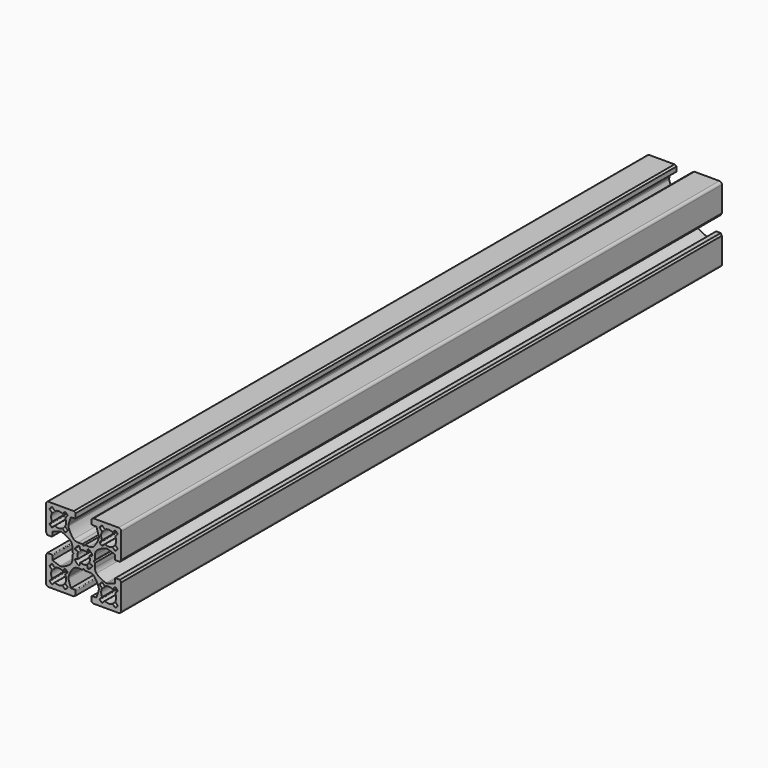
from build123d import *

# Parameters (mm, degrees)
F1_DEPTH = 300


# Not quite as in the source:
# - ends of sketch curves that miss each other by under 0.0002 mm in the source are joined


with BuildPart() as f1:
    # F0 (on Front) → F1 (new body)
    with BuildSketch(Plane.XZ):
        with BuildLine():
            Line((-10.317882, -28.053804), (-8.817882, -28.053804))
            Line((-8.817882, -28.053804), (-8.317882, -27.553804))
            Line((-8.317882, -27.553804), (-8.317882, -25.835963))
            ThreePointArc((-8.317882, -25.835963), (-8.1666472628, -24.8954650055), (-7.7281910149, -24.049790989))
            ThreePointArc((-7.7281910149, -24.049790989), (-5.9278016138, -22.7791417483), (-3.8900220756, -21.9404487353))
            ThreePointArc((-3.8900220756, -21.9404487353), (-3.6281322729, -21.9188378518), (-3.3696549943, -21.9661959825))
            Line((-3.3696549943, -21.9661959825), (-0.317882, -22.953804))
            Line((-0.317882, -22.953804), (-0.317882, -24.603804))
            ThreePointArc((-0.317882, -24.603804), (-0.2300140344, -24.8159360344), (-0.017882, -24.903804))
            Line((-0.017882, -24.903804), (1.682118, -24.903804))
            Line((1.682118, -24.903804), (2.182118, -24.103804))
            Line((2.182118, -24.103804), (2.182118, -14.053804))
            ThreePointArc((2.182118, -14.053804), (1.8892247812, -13.3466972188), (1.182118, -13.053804))
            Line((1.182118, -13.053804), (-8.867882, -13.053804))
            Line((-8.867882, -13.053804), (-9.667882, -13.553804))
            Line((-9.667882, -13.553804), (-9.667882, -15.253804))
            ThreePointArc((-9.667882, -15.253804), (-9.5800140344, -15.4659360344), (-9.367882, -15.553804))
            Line((-9.367882, -15.553804), (-7.717882, -15.553804))
            Line((-7.717882, -15.553804), (-6.730274, -18.605577))
            ThreePointArc((-6.730274, -18.605577), (-6.6829159047, -18.8640542036), (-6.7045263914, -19.1259439149))
            ThreePointArc((-6.7045263914, -19.1259439149), (-7.5432189083, -21.1637239049), (-8.8138685119, -22.9641134339))
            ThreePointArc((-8.8138685119, -22.9641134339), (-9.6595430055, -23.4025692628), (-10.600041, -23.553804))
            Line((-10.600041, -23.553804), (-12.317882, -23.553804))
            Line((-12.317882, -23.553804), (-12.817882, -24.053804))
            Line((-12.817882, -24.053804), (-12.817882, -25.553804))
            ThreePointArc((-12.817882, -25.553804), (-12.2892723342, -25.6103286428), (-11.7845662465, -25.777346543))
            ThreePointArc((-11.7845662465, -25.777346543), (-11.521192295, -25.7698304515), (-11.3653270693, -25.5573959875))
            Line((-11.3653270693, -25.5573959875), (-11.231756, -24.816462))
            ThreePointArc((-11.231756, -24.816462), (-11.061392872, -24.5969122529), (-10.7838767336, -24.6114195492))
            ThreePointArc((-10.7838767336, -24.6114195492), (-9.990624391, -25.2265473595), (-9.3754974572, -26.0198002702))
            ThreePointArc((-9.3754974572, -26.0198002702), (-9.3609903588, -26.2973161033), (-9.5805400125, -26.4676789307))
            Line((-9.5805400125, -26.4676789307), (-10.321473, -26.601249))
            ThreePointArc((-10.321473, -26.601249), (-10.5339073555, -26.757114112), (-10.5414238716, -27.0204879417))
            ThreePointArc((-10.5414238716, -27.0204879417), (-10.3744066428, -27.5251943342), (-10.317882, -28.053804))
        make_face()
        with BuildLine():
            ThreePointArc((-5.5627339656, -19.7356560344), (-5.4787894201, -19.5718836819), (-5.5062620121, -19.389913006))
            ThreePointArc((-5.5062620121, -19.389913006), (-5.820221, -18.053804), (-5.5062614757, -16.7176952608))
            ThreePointArc((-5.5062614757, -16.7176952608), (-5.4787894201, -16.5357243181), (-5.5627339656, -16.3719519656))
            Line((-5.5627339656, -16.3719519656), (-6.303305, -15.631381))
            ThreePointArc((-6.303305, -15.631381), (-6.3907399595, -15.4353436467), (-6.3248118511, -15.2310671199))
            ThreePointArc((-6.3248118511, -15.2310671199), (-6.0022020125, -14.8718239818), (-5.6429589383, -14.5492140766))
            ThreePointArc((-5.6429589383, -14.5492140766), (-5.4386817022, -14.4832850218), (-5.2426439656, -14.5707209656))
            Line((-5.2426439656, -14.5707209656), (-4.502074, -15.311292))
            ThreePointArc((-4.502074, -15.311292), (-4.3383016819, -15.3952365799), (-4.156331006, -15.3677639879))
            ThreePointArc((-4.156331006, -15.3677639879), (-2.8202214477, -15.053804), (-1.484111862, -15.3677637227))
            ThreePointArc((-1.484111862, -15.3677637227), (-1.3021413181, -15.3952365799), (-1.1383689656, -15.3112920344))
            Line((-1.1383689656, -15.3112920344), (-0.397799, -14.570721))
            ThreePointArc((-0.397799, -14.570721), (-0.2017612978, -14.4832850218), (0.0025159751, -14.5492140309))
            ThreePointArc((0.0025159751, -14.5492140309), (0.3617595153, -14.8718234847), (0.684369412, -15.2310666682))
            ThreePointArc((0.684369412, -15.2310666682), (0.7502979573, -15.4353436866), (0.6628620344, -15.6313810344))
            Line((0.6628620344, -15.6313810344), (-0.077709, -16.371952))
            ThreePointArc((-0.077709, -16.371952), (-0.1616535799, -16.5357243181), (-0.1341809879, -16.717694994))
            ThreePointArc((-0.1341809879, -16.717694994), (0.179779, -18.053804), (-0.1341807227, -19.389913138))
            ThreePointArc((-0.1341807227, -19.389913138), (-0.1616535799, -19.5718836819), (-0.0777090344, -19.7356560344))
            Line((-0.0777090344, -19.7356560344), (0.662862, -20.476227))
            ThreePointArc((0.662862, -20.476227), (0.7502979573, -20.6722643134), (0.6843694576, -20.8765413686))
            ThreePointArc((0.6843694576, -20.8765413686), (0.3617595153, -21.2357845153), (0.0025163318, -21.558394412))
            ThreePointArc((0.0025163318, -21.558394412), (-0.2017612978, -21.6243229782), (-0.3977990344, -21.5368870344))
            Line((-0.3977990344, -21.5368870344), (-1.138369, -20.796316))
            ThreePointArc((-1.138369, -20.796316), (-1.3021413181, -20.7123714201), (-1.484111994, -20.7398440121))
            ThreePointArc((-1.484111994, -20.7398440121), (-2.8202214477, -21.053804), (-4.1563309396, -20.7398438786))
            ThreePointArc((-4.1563309396, -20.7398438786), (-4.3383016819, -20.7123714201), (-4.5020740344, -20.7963159656))
            Line((-4.5020740344, -20.7963159656), (-5.242644, -21.536887))
            ThreePointArc((-5.242644, -21.536887), (-5.4386817022, -21.6243229782), (-5.6429589751, -21.5583939691))
            ThreePointArc((-5.6429589751, -21.5583939691), (-6.0022020125, -21.2357840182), (-6.3248118054, -20.8765408433))
            ThreePointArc((-6.3248118054, -20.8765408433), (-6.3907399595, -20.6722643533), (-6.3033045344, -20.4762274656))
            Line((-6.3033045344, -20.4762274656), (-5.5627339656, -19.7356560344))
        make_face(mode=Mode.SUBTRACT)
        with BuildLine():
            Line((-16.817882, -28.053804), (-15.317882, -28.053804))
            ThreePointArc((-15.317882, -28.053804), (-15.2613573135, -27.5251941322), (-15.0943392862, -27.0204878701))
            ThreePointArc((-15.0943392862, -27.0204878701), (-15.1018556445, -26.757114112), (-15.3142900125, -26.6012490693))
            Line((-15.3142900125, -26.6012490693), (-16.055223, -26.467679))
            ThreePointArc((-16.055223, -26.467679), (-16.2747726412, -26.2973161033), (-16.2602657097, -26.0198001716))
            ThreePointArc((-16.2602657097, -26.0198001716), (-15.6451391247, -25.2265468753), (-14.8518861678, -24.611419716))
            ThreePointArc((-14.8518861678, -24.611419716), (-14.574370128, -24.5969122529), (-14.4040070693, -24.8164620125))
            Line((-14.4040070693, -24.8164620125), (-14.270436, -25.557396))
            ThreePointArc((-14.270436, -25.557396), (-14.114570705, -25.7698304515), (-13.8511966819, -25.7773467007))
            ThreePointArc((-13.8511966819, -25.7773467007), (-13.3464912208, -25.6103285465), (-12.817882, -25.553804))
            Line((-12.817882, -25.553804), (-12.817882, -24.053804))
            Line((-12.817882, -24.053804), (-13.317882, -23.553804))
            Line((-13.317882, -23.553804), (-15.035723, -23.553804))
            ThreePointArc((-15.035723, -23.553804), (-15.9762206131, -23.4025693887), (-16.8218943655, -22.9641134932))
            ThreePointArc((-16.8218943655, -22.9641134932), (-18.0925440917, -21.1637239049), (-18.9312372647, -19.1259440756))
            ThreePointArc((-18.9312372647, -19.1259440756), (-18.952848093, -18.864054156), (-18.9054896298, -18.6055767962))
            Line((-18.9054896298, -18.6055767962), (-17.917882, -15.553804))
            Line((-17.917882, -15.553804), (-16.267882, -15.553804))
            ThreePointArc((-16.267882, -15.553804), (-16.0557499656, -15.4659360344), (-15.967882, -15.253804))
            Line((-15.967882, -15.253804), (-15.967882, -13.553804))
            Line((-15.967882, -13.553804), (-16.767882, -13.053804))
            Line((-16.767882, -13.053804), (-26.817882, -13.053804))
            ThreePointArc((-26.817882, -13.053804), (-27.5249887812, -13.3466972188), (-27.817882, -14.053804))
            Line((-27.817882, -14.053804), (-27.817882, -24.103804))
            Line((-27.817882, -24.103804), (-27.317882, -24.903804))
            Line((-27.317882, -24.903804), (-25.617882, -24.903804))
            ThreePointArc((-25.617882, -24.903804), (-25.4057499656, -24.8159360344), (-25.317882, -24.603804))
            Line((-25.317882, -24.603804), (-25.317882, -22.953804))
            Line((-25.317882, -22.953804), (-22.266108, -21.966196))
            ThreePointArc((-22.266108, -21.966196), (-22.0076307271, -21.9188378518), (-21.7457409226, -21.9404486442))
            ThreePointArc((-21.7457409226, -21.9404486442), (-19.7079616374, -22.7791421598), (-17.907572504, -24.049791567))
            ThreePointArc((-17.907572504, -24.049791567), (-17.4691166439, -24.8954652882), (-17.317882, -25.835963))
            Line((-17.317882, -25.835963), (-17.317882, -27.553804))
            Line((-17.317882, -27.553804), (-16.817882, -28.053804))
        make_face()
        with BuildLine():
            ThreePointArc((-20.1318415243, -16.7176952608), (-19.817882, -18.053804), (-20.1318415243, -19.3899127392))
            ThreePointArc((-20.1318415243, -19.3899127392), (-20.1593135799, -19.5718836819), (-20.0753690344, -19.7356560344))
            Line((-20.0753690344, -19.7356560344), (-19.334799, -20.476227))
            ThreePointArc((-19.334799, -20.476227), (-19.2473630595, -20.6722640002), (-19.3132911489, -20.8765408801))
            ThreePointArc((-19.3132911489, -20.8765408801), (-19.6359009875, -21.2357840182), (-19.9951440617, -21.5583939234))
            ThreePointArc((-19.9951440617, -21.5583939234), (-20.1994212978, -21.6243229782), (-20.3954590344, -21.5368870344))
            Line((-20.3954590344, -21.5368870344), (-21.136029, -20.796316))
            ThreePointArc((-21.136029, -20.796316), (-21.2998015274, -20.7123715492), (-21.4817721923, -20.7398436134))
            ThreePointArc((-21.4817721923, -20.7398436134), (-22.8178815523, -21.053804), (-24.153991138, -20.7398442773))
            ThreePointArc((-24.153991138, -20.7398442773), (-24.3359616819, -20.7123714201), (-24.4997340344, -20.7963159656))
            Line((-24.4997340344, -20.7963159656), (-25.240304, -21.536887))
            ThreePointArc((-25.240304, -21.536887), (-25.4363417022, -21.6243229782), (-25.6406189751, -21.5583939691))
            ThreePointArc((-25.6406189751, -21.5583939691), (-25.9998625153, -21.2357845153), (-26.322472412, -20.8765413318))
            ThreePointArc((-26.322472412, -20.8765413318), (-26.3884009573, -20.6722643134), (-26.3009650344, -20.4762269656))
            Line((-26.3009650344, -20.4762269656), (-25.560394, -19.735656))
            ThreePointArc((-25.560394, -19.735656), (-25.4764494201, -19.5718836819), (-25.5039220121, -19.389913006))
            ThreePointArc((-25.5039220121, -19.389913006), (-25.817882, -18.053804), (-25.5039222773, -16.717694862))
            ThreePointArc((-25.5039222773, -16.717694862), (-25.4764494201, -16.5357243181), (-25.5603939656, -16.3719519656))
            Line((-25.5603939656, -16.3719519656), (-26.300965, -15.631381))
            ThreePointArc((-26.300965, -15.631381), (-26.3884009573, -15.4353436866), (-26.3224724576, -15.2310666314))
            ThreePointArc((-26.3224724576, -15.2310666314), (-25.9998625153, -14.8718234847), (-25.6406193318, -14.549213588))
            ThreePointArc((-25.6406193318, -14.549213588), (-25.4363417022, -14.4832850218), (-25.2403039656, -14.5707209656))
            Line((-25.2403039656, -14.5707209656), (-24.499734, -15.311292))
            ThreePointArc((-24.499734, -15.311292), (-24.3359616819, -15.3952365799), (-24.153991006, -15.3677639879))
            ThreePointArc((-24.153991006, -15.3677639879), (-22.8178815523, -15.053804), (-21.4817720604, -15.3677641214))
            ThreePointArc((-21.4817720604, -15.3677641214), (-21.2998015274, -15.3952364508), (-21.1360294656, -15.3112915344))
            Line((-21.1360294656, -15.3112915344), (-20.395459, -14.570721))
            ThreePointArc((-20.395459, -14.570721), (-20.1994212978, -14.4832850218), (-19.9951440249, -14.5492140309))
            ThreePointArc((-19.9951440249, -14.5492140309), (-19.6359009875, -14.8718239818), (-19.3132911946, -15.2310671567))
            ThreePointArc((-19.3132911946, -15.2310671567), (-19.2473630595, -15.4353439998), (-19.3347989656, -15.6313810344))
            Line((-19.3347989656, -15.6313810344), (-20.075369, -16.371952))
            ThreePointArc((-20.075369, -16.371952), (-20.1593135799, -16.5357243181), (-20.1318415243, -16.7176952608))
        make_face(mode=Mode.SUBTRACT)
        with BuildLine():
            Line((-8.317882, -28.553804), (-8.817882, -28.053804))
            Line((-8.817882, -28.053804), (-10.317882, -28.053804))
            ThreePointArc((-10.317882, -28.053804), (-10.3744066428, -28.5824136658), (-10.541424543, -29.0871197535))
            ThreePointArc((-10.541424543, -29.0871197535), (-10.5339073967, -29.3504938095), (-10.3214731621, -29.5063588992))
            Line((-10.3214731621, -29.5063588992), (-9.58054, -29.639929))
            ThreePointArc((-9.58054, -29.639929), (-9.3609903588, -29.8102918967), (-9.3754972903, -30.0878078284))
            ThreePointArc((-9.3754972903, -30.0878078284), (-9.990624391, -30.8810606405), (-10.783877091, -31.496187846))
            ThreePointArc((-10.783877091, -31.496187846), (-11.061392872, -31.5106957471), (-11.2317559307, -31.2911459875))
            Line((-11.2317559307, -31.2911459875), (-11.365327, -30.550212))
            ThreePointArc((-11.365327, -30.550212), (-11.521192112, -30.3377776445), (-11.7845659417, -30.3302611284))
            ThreePointArc((-11.7845659417, -30.3302611284), (-12.2892721322, -30.4972793135), (-12.817882, -30.553804))
            Line((-12.817882, -30.553804), (-12.817882, -32.053804))
            Line((-12.817882, -32.053804), (-12.317882, -32.553804))
            Line((-12.317882, -32.553804), (-10.600041, -32.553804))
            ThreePointArc((-10.600041, -32.553804), (-9.6595430055, -32.7050387372), (-8.813868989, -33.1434949851))
            ThreePointArc((-8.813868989, -33.1434949851), (-7.5432189083, -34.9438840951), (-6.7045257353, -36.9816639244))
            ThreePointArc((-6.7045257353, -36.9816639244), (-6.6829158812, -37.2435533212), (-6.7302739825, -37.5020300057))
            Line((-6.7302739825, -37.5020300057), (-7.717882, -40.553804))
            Line((-7.717882, -40.553804), (-9.367882, -40.553804))
            ThreePointArc((-9.367882, -40.553804), (-9.5800140344, -40.6416719656), (-9.667882, -40.853804))
            Line((-9.667882, -40.853804), (-9.667882, -42.553804))
            Line((-9.667882, -42.553804), (-8.867882, -43.053804))
            Line((-8.867882, -43.053804), (1.182118, -43.053804))
            ThreePointArc((1.182118, -43.053804), (1.8892247812, -42.7609107812), (2.182118, -42.053804))
            Line((2.182118, -42.053804), (2.182118, -32.003804))
            Line((2.182118, -32.003804), (1.682118, -31.203804))
            Line((1.682118, -31.203804), (-0.017882, -31.203804))
            ThreePointArc((-0.017882, -31.203804), (-0.2300140344, -31.2916719656), (-0.317882, -31.503804))
            Line((-0.317882, -31.503804), (-0.317882, -33.153804))
            Line((-0.317882, -33.153804), (-3.369655, -34.141412))
            ThreePointArc((-3.369655, -34.141412), (-3.6281322729, -34.1887701482), (-3.8900220774, -34.1671593558))
            ThreePointArc((-3.8900220774, -34.1671593558), (-5.9278016138, -33.3284662517), (-7.7281909374, -32.0578169295))
            ThreePointArc((-7.7281909374, -32.0578169295), (-8.1666472628, -31.2121429945), (-8.317882, -30.271645))
            Line((-8.317882, -30.271645), (-8.317882, -28.553804))
        make_face()
        with BuildLine():
            ThreePointArc((-5.507146239, -39.3904841188), (-5.8210019909, -38.0543501064), (-5.5069379006, -36.7182650494))
            ThreePointArc((-5.5069379006, -36.7182650494), (-5.4794506299, -36.5362965287), (-5.5633824662, -36.3725174663))
            Line((-5.5633824662, -36.3725174663), (-6.303896, -35.631889))
            ThreePointArc((-6.303896, -35.631889), (-6.3913162338, -35.4358449105), (-6.3253716664, -35.2315732687))
            ThreePointArc((-6.3253716664, -35.2315732687), (-6.0027340882, -34.8723550769), (-5.6434657786, -34.5497732749))
            ThreePointArc((-5.6434657786, -34.5497732749), (-5.4391833549, -34.483860277), (-5.2431524662, -34.5713114663))
            Line((-5.2431524662, -34.5713114663), (-4.50264, -35.31194))
            ThreePointArc((-4.50264, -35.31194), (-4.3388740212, -35.3958977668), (-4.1569008286, -35.3684393446))
            ThreePointArc((-4.1569008286, -35.3684393446), (-2.8207674361, -35.0545840092), (-1.4846830494, -35.3686480994))
            ThreePointArc((-1.4846830494, -35.3686480994), (-1.3027146578, -35.3961343911), (-1.1389359663, -35.3122030337))
            Line((-1.1389359663, -35.3122030337), (-0.398307, -34.57169))
            ThreePointArc((-0.398307, -34.57169), (-0.2022626922, -34.4842688081), (0.0020096134, -34.5502132386))
            ThreePointArc((0.0020096134, -34.5502132386), (0.3612269231, -34.8728519118), (0.6838087251, -35.2321202214))
            ThreePointArc((0.6838087251, -35.2321202214), (0.7497216831, -35.4364023869), (0.6622700337, -35.6324330337))
            Line((0.6622700337, -35.6324330337), (-0.078358, -36.372946))
            ThreePointArc((-0.078358, -36.372946), (-0.1623158238, -36.5367113277), (-0.1348573446, -36.7186841714))
            ThreePointArc((-0.1348573446, -36.7186841714), (0.1789979909, -38.0548178935), (-0.1350659009, -39.3909025518))
            ThreePointArc((-0.1350659009, -39.3909025518), (-0.162552241, -39.5728712621), (-0.0786200338, -39.7366500338))
            Line((-0.0786200338, -39.7366500338), (0.661893, -40.477278))
            ThreePointArc((0.661893, -40.477278), (0.7493132149, -40.6733227364), (0.6833686664, -40.8775947313))
            ThreePointArc((0.6833686664, -40.8775947313), (0.3607308072, -41.2368122042), (0.0014628737, -41.5593938432))
            ThreePointArc((0.0014628737, -41.5593938432), (-0.202819292, -41.625306742), (-0.3988500338, -41.5378560338))
            Line((-0.3988500338, -41.5378560338), (-1.139363, -40.797227))
            ThreePointArc((-1.139363, -40.797227), (-1.303129108, -40.7132702121), (-1.4851017727, -40.7407284571))
            ThreePointArc((-1.4851017727, -40.7407284571), (-2.8212354459, -41.0545839909), (-4.157320149, -40.7405202994))
            ThreePointArc((-4.157320149, -40.7405202994), (-4.3392886912, -40.7130336658), (-4.5030675338, -40.7969654663))
            Line((-4.5030675338, -40.7969654663), (-5.243696, -41.537478))
            ThreePointArc((-5.243696, -41.537478), (-5.4397403476, -41.624898194), (-5.6440121248, -41.5589541549))
            ThreePointArc((-5.6440121248, -41.5589541549), (-6.0032304261, -41.2363165853), (-6.3258123317, -40.8770482671))
            ThreePointArc((-6.3258123317, -40.8770482671), (-6.3917246831, -40.6727656131), (-6.3042730337, -40.4767349663))
            Line((-6.3042730337, -40.4767349663), (-5.563645, -39.736222))
            ThreePointArc((-5.563645, -39.736222), (-5.4796873054, -39.5724564631), (-5.507146239, -39.3904841188))
        make_face(mode=Mode.SUBTRACT)
        with BuildLine():
            ThreePointArc((-15.0943392862, -29.0871201299), (-15.2613573135, -28.5824138678), (-15.317882, -28.053804))
            Line((-15.317882, -28.053804), (-16.817882, -28.053804))
            Line((-16.817882, -28.053804), (-17.317882, -28.553804))
            Line((-17.317882, -28.553804), (-17.317882, -30.271645))
            ThreePointArc((-17.317882, -30.271645), (-17.4691166439, -31.2121427118), (-17.9075726307, -32.0578165326))
            ThreePointArc((-17.9075726307, -32.0578165326), (-19.7079616374, -33.3284658402), (-21.7457409999, -34.1671590005))
            ThreePointArc((-21.7457409999, -34.1671590005), (-22.0076307271, -34.1887701482), (-22.2661080057, -34.1414120175))
            Line((-22.2661080057, -34.1414120175), (-25.317882, -33.153804))
            Line((-25.317882, -33.153804), (-25.317882, -31.503804))
            ThreePointArc((-25.317882, -31.503804), (-25.4057499656, -31.2916719656), (-25.617882, -31.203804))
            Line((-25.617882, -31.203804), (-27.317882, -31.203804))
            Line((-27.317882, -31.203804), (-27.817882, -32.003804))
            Line((-27.817882, -32.003804), (-27.817882, -42.053804))
            ThreePointArc((-27.817882, -42.053804), (-27.5249887812, -42.7609107812), (-26.817882, -43.053804))
            Line((-26.817882, -43.053804), (-16.767882, -43.053804))
            Line((-16.767882, -43.053804), (-15.967882, -42.553804))
            Line((-15.967882, -42.553804), (-15.967882, -40.853804))
            ThreePointArc((-15.967882, -40.853804), (-16.0557499656, -40.6416719656), (-16.267882, -40.553804))
            Line((-16.267882, -40.553804), (-17.917882, -40.553804))
            Line((-17.917882, -40.553804), (-18.905489, -37.50203))
            ThreePointArc((-18.905489, -37.50203), (-18.9528481165, -37.2435533689), (-18.9312375634, -36.9816638775))
            ThreePointArc((-18.9312375634, -36.9816638775), (-18.0925440917, -34.9438840951), (-16.8218944881, -33.1434945661))
            ThreePointArc((-16.8218944881, -33.1434945661), (-15.9762206131, -32.7050386113), (-15.035723, -32.553804))
            Line((-15.035723, -32.553804), (-13.317882, -32.553804))
            Line((-13.317882, -32.553804), (-12.817882, -32.053804))
            Line((-12.817882, -32.053804), (-12.817882, -30.553804))
            ThreePointArc((-12.817882, -30.553804), (-13.3464914228, -30.4972794098), (-13.8511973007, -30.3302616625))
            ThreePointArc((-13.8511973007, -30.3302616625), (-14.114570888, -30.3377776445), (-14.2704359307, -30.5502120125))
            Line((-14.2704359307, -30.5502120125), (-14.404007, -31.291146))
            ThreePointArc((-14.404007, -31.291146), (-14.574370128, -31.5106957471), (-14.8518862664, -31.4961884508))
            ThreePointArc((-14.8518862664, -31.4961884508), (-15.6451391247, -30.8810611247), (-16.260266284, -30.0878081678))
            ThreePointArc((-16.260266284, -30.0878081678), (-16.2747726412, -29.8102918967), (-16.0552229875, -29.6399290693))
            Line((-16.0552229875, -29.6399290693), (-15.31429, -29.506358))
            ThreePointArc((-15.31429, -29.506358), (-15.1018556033, -29.3504938095), (-15.0943392862, -29.0871201299))
        make_face()
        with BuildLine():
            ThreePointArc((-20.0747205338, -36.3725174663), (-20.1586523342, -36.5362963089), (-20.1311656295, -36.7182648157))
            ThreePointArc((-20.1311656295, -36.7182648157), (-19.8171020091, -38.0543498837), (-20.1309575628, -39.3904837201))
            ThreePointArc((-20.1309575628, -39.3904837201), (-20.1584156946, -39.5724564631), (-20.0744580337, -39.7362220337))
            Line((-20.0744580337, -39.7362220337), (-19.33383, -40.476735))
            ThreePointArc((-19.33383, -40.476735), (-19.2463783169, -40.6727656131), (-19.3122908476, -40.8770481227))
            ThreePointArc((-19.3122908476, -40.8770481227), (-19.6348730769, -41.2363160882), (-19.9940910142, -41.5589539824))
            ThreePointArc((-19.9940910142, -41.5589539824), (-20.1983629105, -41.6248982338), (-20.3944070337, -41.5374780337))
            Line((-20.3944070337, -41.5374780337), (-21.135036, -40.796965))
            ThreePointArc((-21.135036, -40.796965), (-21.2988146578, -40.7130336089), (-21.4807828157, -40.7405203705))
            ThreePointArc((-21.4807828157, -40.7405203705), (-22.8168676587, -41.0545839908), (-24.1530013171, -40.7407286377))
            ThreePointArc((-24.1530013171, -40.7407286377), (-24.334973892, -40.7132702121), (-24.4987395337, -40.7972274662))
            Line((-24.4987395337, -40.7972274662), (-25.239253, -41.537856))
            ThreePointArc((-25.239253, -41.537856), (-25.435283708, -41.625306742), (-25.6395657293, -41.5593936639))
            ThreePointArc((-25.6395657293, -41.5593936639), (-25.99883431, -41.2368127014), (-26.3214719824, -40.8775949858))
            ThreePointArc((-26.3214719824, -40.8775949858), (-26.3874162149, -40.6733227364), (-26.2999955337, -40.4772784662))
            Line((-26.2999955337, -40.4772784662), (-25.559483, -39.73665))
            ThreePointArc((-25.559483, -39.73665), (-25.475550759, -39.5728712621), (-25.5030371701, -39.3909025871))
            ThreePointArc((-25.5030371701, -39.3909025871), (-25.8171019909, -38.0548178936), (-25.503246239, -36.7186838812))
            ThreePointArc((-25.503246239, -36.7186838812), (-25.4757871762, -36.5367113277), (-25.5597444663, -36.3729454662))
            Line((-25.5597444663, -36.3729454662), (-26.300374, -35.632433))
            ThreePointArc((-26.300374, -35.632433), (-26.3878247021, -35.4364020339), (-26.3219121524, -35.2321198773))
            ThreePointArc((-26.3219121524, -35.2321198773), (-25.9993304261, -34.8728514147), (-25.6401123794, -34.550213529))
            ThreePointArc((-25.6401123794, -34.550213529), (-25.4358403078, -34.4842688081), (-25.2397959662, -34.5716899662))
            Line((-25.2397959662, -34.5716899662), (-24.499168, -35.312203))
            ThreePointArc((-24.499168, -35.312203), (-24.3353886912, -35.3961343342), (-24.1534201843, -35.3686476295))
            ThreePointArc((-24.1534201843, -35.3686476295), (-22.8173356686, -35.0545840091), (-21.4812022799, -35.3684395628))
            ThreePointArc((-21.4812022799, -35.3684395628), (-21.2992289788, -35.3958977668), (-21.1354629663, -35.3119400337))
            Line((-21.1354629663, -35.3119400337), (-20.39495, -34.571312))
            ThreePointArc((-20.39495, -34.571312), (-20.1989200339, -34.4838602979), (-19.9946378773, -34.5497728476))
            ThreePointArc((-19.9946378773, -34.5497728476), (-19.63536969, -34.8723552987), (-19.312731624, -35.2315735027))
            ThreePointArc((-19.312731624, -35.2315735027), (-19.2467867662, -35.4358449105), (-19.3342069663, -35.6318890337))
            Line((-19.3342069663, -35.6318890337), (-20.0747205338, -36.3725174663))
        make_face(mode=Mode.SUBTRACT)
    extrude(amount=F1_DEPTH)


solid = f1.part
